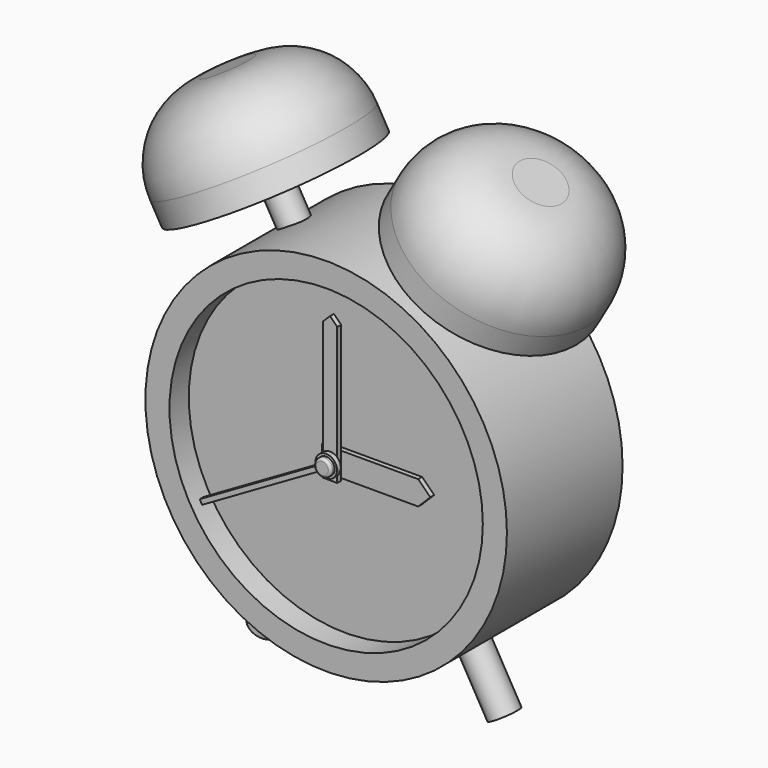
from build123d import *

# Parameters (mm, degrees)
F0_R      = 75
F1_DEPTH  = 60
F2_R      = 65
F3_DEPTH  = 10
F7_R      = 30
F8_ANGLE  = 30
F9_ANGLE  = 300
F10_R     = 2
F11_DEPTH = 4
F12_W     = 45
F12_H     = 10
F12_R     = 2
F13_DEPTH = 2
F14_SIZE  = 4.99999
F15_W     = 6
F15_H     = 49
F15_H_2   = 10
F15_H_3   = 1
F16_DEPTH = 2
F17_SIZE  = 2.99999
F18_W     = 2
F18_H     = 54
F19_DEPTH = 2
F20_ANGLE = 300
F21_R     = 3.5
F22_DEPTH = 2
F23_R     = 1


# Not quite as in the source:
# - a fillet or chamfer is up to 0.001 mm smaller than in the source, because OpenCascade refuses the exact size


with BuildPart() as f1:
    # F0 (on Front) → F1 (new body)
    with BuildSketch(Plane.XZ):
        Circle(F0_R)
    extrude(amount=-F1_DEPTH)

    # F2 (on face) → F3 (cut)
    with BuildSketch(Plane.XZ):
        Circle(F2_R)
    extrude(amount=-F3_DEPTH, mode=Mode.SUBTRACT)


with BuildPart() as f5:
    # F4 (on face) → F5 (revolve)
    with BuildSketch(Plane.XZ.offset(-10)):
        with BuildLine():
            Line((0, 130), (0, 65))
            ThreePointArc((0, 65), (3.0032072378, 64.9305840593), (6, 64.7224845011))
            Line((6, 64.7224845011), (6, 90))
            Line((6, 90), (40, 90))
            Line((40, 90), (40, 130))
            Line((40, 130), (0, 130))
        make_face()
        with BuildLine():
            Line((0, 65), (0, 0))
            Line((0, 0), (0, -65))
            ThreePointArc((0, -65), (3.0032072378, -64.9305840593), (6, -64.7224845011))
            Line((6, -64.7224845011), (6, 64.7224845011))
            ThreePointArc((6, 64.7224845011), (3.0032072378, 64.9305840593), (0, 65))
        make_face()
        with BuildLine():
            ThreePointArc((6, -64.7224845011), (3.0032072378, -64.9305840593), (0, -65))
            Line((0, -65), (0, -100))
            Line((0, -100), (6, -100))
            Line((6, -100), (6, -64.7224845011))
        make_face()
    revolve(axis=Axis((0, 10, 65), (0, 0, 1)))


with BuildPart() as f5_1:
    # F6: moved
    add(f5.part.moved(Location((0, 20, 0))))

    # F7
    f7_edges = [f5_1.edges().sort_by_distance(p)[0] for p in [
        (-40, 30, 130),
    ]]
    fillet(f7_edges, radius=F7_R)


with BuildPart() as f5_2:
    # F8: moved
    add(f5_1.part.rotate(Axis((0, 0, 0), (0, -1, 0)), F8_ANGLE))


with BuildPart() as f9_1:
    # F9: copy of F5
    add(f5_2.part.rotate(Axis((0, 0, 0), (0, -1, 0)), F9_ANGLE))


with BuildPart() as f11:
    # F10 (on face) → F11 (new body)
    with BuildSketch(Plane.XZ.offset(-10)):
        Circle(F10_R)
    extrude(amount=F11_DEPTH)


with BuildPart() as f13:
    # F12 (on face) → F13 (new body)
    with BuildSketch(Plane.XZ.offset(-6)):
        with Locations((17.5, 0)):
            Rectangle(F12_W, F12_H)
        Circle(F12_R, mode=Mode.SUBTRACT)
        Circle(F12_R)
    extrude(amount=F13_DEPTH)

    # F14 (size 5 in the source; OpenCascade refuses exactly that, so slightly less here)
    f14_edges = [f13.edges().sort_by_distance(p)[0] for p in [
        (40, 5, 5),
        (40, 5, -5),
    ]]
    chamfer(f14_edges, length=F14_SIZE)


with BuildPart() as f16:
    # F15 (on face) → F16 (new body)
    with BuildSketch(Plane.XZ.offset(-4)):
        with Locations((0, 29.5)):
            Rectangle(F15_W, F15_H)
        Rectangle(F15_W, F15_H_2)
        with Locations((0, -5.5)):
            Rectangle(F15_W, F15_H_3)
    extrude(amount=F16_DEPTH)

    # F17 (size 3 in the source; OpenCascade refuses exactly that, so slightly less here)
    f17_edges = [f16.edges().sort_by_distance(p)[0] for p in [
        (3, 3, 54),
        (-3, 3, 54),
    ]]
    chamfer(f17_edges, length=F17_SIZE)


with BuildPart() as f19:
    # F18 (on face) → F19 (new body)
    with BuildSketch(Plane.XZ.offset(-2)):
        with BuildLine():
            Line((1, -6), (1, -4.3874821937))
            ThreePointArc((1, -4.3874821937), (2.0656642209, -3.9978783531), (3, -3.3541019662))
            Line((3, -3.3541019662), (3, 3.3541019662))
            ThreePointArc((3, 3.3541019662), (0, 4.5), (-3, 3.3541019662))
            Line((-3, 3.3541019662), (-3, -3.3541019662))
            ThreePointArc((-3, -3.3541019662), (-2.0656642209, -3.9978783531), (-1, -4.3874821937))
            Line((-1, -4.3874821937), (-1, -6))
            Line((-1, -6), (1, -6))
        make_face()
        with BuildLine():
            Line((3, 3.3541019662), (3, -3.3541019662))
            ThreePointArc((3, -3.3541019662), (4.5, 0), (3, 3.3541019662))
        make_face()
        with Locations((0, -33)):
            Rectangle(F18_W, F18_H)
        with BuildLine():
            Line((-3, -3.3541019662), (-3, 3.3541019662))
            ThreePointArc((-3, 3.3541019662), (-4.5, 0), (-3, -3.3541019662))
        make_face()
    extrude(amount=F19_DEPTH)


with BuildPart() as f19_1:
    # F20: moved
    add(f19.part.rotate(Axis((0, 0, 0), (0, -1, 0)), F20_ANGLE))


with BuildPart() as f22:
    # F21 (on face) → F22 (new body)
    with BuildSketch(Plane.XZ):
        Circle(F21_R)
    extrude(amount=F22_DEPTH)

    # F23
    f23_edges = [f22.edges().sort_by_distance(p)[0] for p in [
        (-3.5, -2, 0),
    ]]
    fillet(f23_edges, radius=F23_R)


solid = Compound([f1.part, f5_2.part, f9_1.part, f11.part, f13.part, f16.part, f19_1.part, f22.part])
